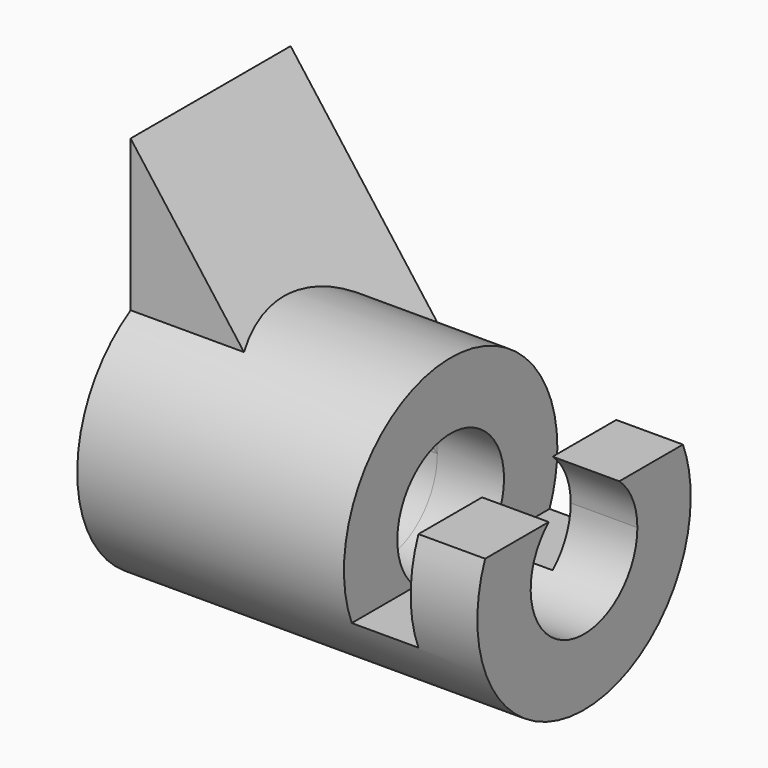
from build123d import *
from build123d import SkipClean  # not in build123d's __all__

# Parameters (mm, degrees)
F0_R          = 25.4
F0_R_2        = 12.7
F1_DEPTH      = 76.2
F3_DEPTH      = 25.4
F5_DEPTH      = 12.7
F5_DEPTH_BACK = 25.4
F6_R          = 12.7
F7_DEPTH      = 38.1


with BuildPart() as f1:
    # F0 (on Right) → F1 (new body)
    with BuildSketch(Plane.YZ):
        Circle(F0_R)
        Circle(F0_R_2, mode=Mode.SUBTRACT)
    extrude(amount=F1_DEPTH)

    # F2 (on Front) → F3 (cut, symmetric)
    with BuildSketch(Plane.XZ):
        Polygon((76.2, 9.525), (76.2, 25.4), (50.8, 25.4), (50.8, -9.525), (63.5, -9.525), (63.5, 9.525), align=None)
    extrude(amount=F3_DEPTH, both=True, mode=Mode.SUBTRACT)

    # F4 (on Front) → F5 (join, two sides)
    with BuildSketch(Plane.XZ) as f5_sk:
        Polygon((0, 50.8), (0, 0), (38.1, 0), align=None)
    extrude(amount=F5_DEPTH)
    extrude(f5_sk.sketch, amount=-F5_DEPTH_BACK)

    # F6 (on Right) → F7 (cut)
    with BuildSketch(Plane.YZ):
        Circle(F6_R)
    with SkipClean():  # cleaning this boolean's faces spoils the solid; the shape is the same uncleaned
        extrude(amount=F7_DEPTH, mode=Mode.SUBTRACT)


solid = f1.part
